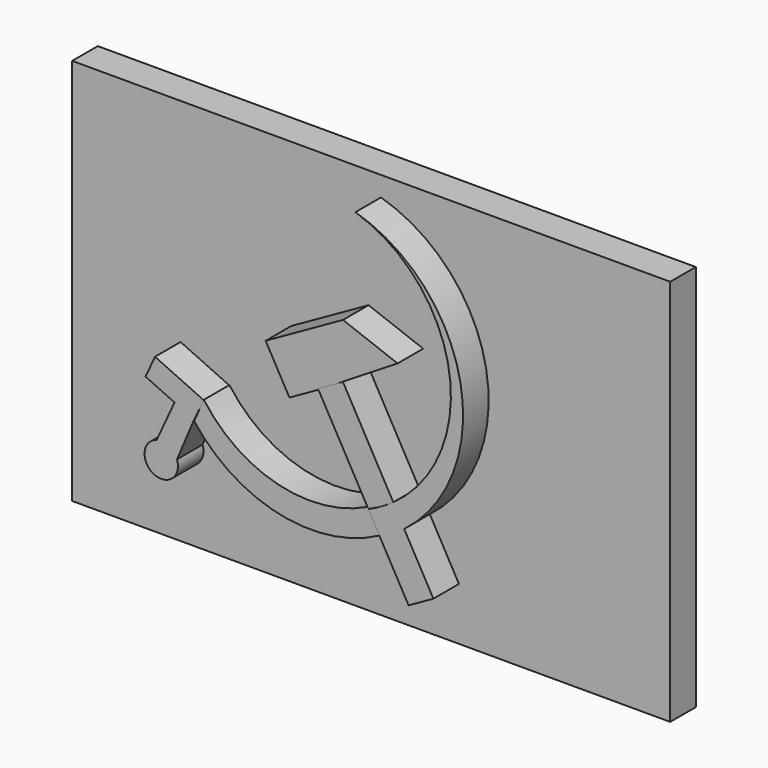
from build123d import *

# Parameters (mm, degrees)
F2_DEPTH = 25.4
F3_W     = 237.6009970903
F3_H     = 153.9654433727
F4_DEPTH = 12.7


with BuildPart() as f2:
    # F0 (on Front) → F2 (new body)
    with BuildSketch(Plane.XZ):
        with BuildLine():
            Line((-64.3306672573, 0), (-71.4252218604, -15.4237253591))
            ThreePointArc((-71.4252218604, -15.4237253591), (-72.6511323462, -27.7185305075), (-63.3521154523, -19.5825994015))
            Line((-63.3521154523, -19.5825994015), (-56.7466728389, -3.9256610908))
            Line((-56.7466728389, -3.9256610908), (-64.3306672573, 0))
        make_face()
        Polygon((-75.8445660615, 5.296125408), (-64.3306672573, 0), (-56.7466728389, -3.9256610908), (-52.6234121387, 4.5160594285), (-72.0855967984, 13.4682112951), align=None)
    extrude(amount=F2_DEPTH)


with BuildPart() as f2b:
    # F0 (on Front) → F2, piece 2 (new body)
    with BuildSketch(Plane.XZ):
        Polygon((-18.6845945711, 16.555041561), (-7.1953465231, 23.0153091252), (24.2997054011, 42.4743108451), (2.6012415412, 50.6354220424), (-28.1310292188, 33.355031617), align=None)
    extrude(amount=F2_DEPTH)


with BuildPart() as f2c:
    # F0 (on Front) → F2, piece 3 (new body)
    with BuildSketch(Plane.XZ):
        with BuildLine():
            ThreePointArc((22.4944953294, -6.7063916159), (17.7171299982, -9.748369789), (12.6509112915, -12.2802226143))
            Line((12.6509112915, -12.2802226143), (17.3099082645, -20.5660051064))
            ThreePointArc((17.3099082645, -20.5660051064), (22.2566100758, -17.7984094918), (26.9180159505, -14.5733917296))
            Line((26.9180159505, -14.5733917296), (22.4944953294, -6.7063916159))
        make_face()
        with BuildLine():
            ThreePointArc((7.5516351178, 89.9414640887), (44.8309857608, 46.2261805414), (22.4944953294, -6.7063916159))
            Line((22.4944953294, -6.7063916159), (26.9180159505, -14.5733917296))
            ThreePointArc((26.9180159505, -14.5733917296), (49.3174772695, 43.6288834146), (7.5516351178, 89.9414640887))
        make_face()
        with BuildLine():
            ThreePointArc((26.9180159505, -14.5733917296), (22.2566100758, -17.7984094918), (17.3099082645, -20.5660051064))
            Line((17.3099082645, -20.5660051064), (28.6526773125, -40.7385267317))
            Line((28.6526773125, -40.7385267317), (38.5128803721, -35.1942517944))
            Line((38.5128803721, -35.1942517944), (26.9180159505, -14.5733917296))
        make_face()
    extrude(amount=F2_DEPTH)


with BuildPart() as f2d:
    # F1 (on Front) → F2, piece 4 (new body)
    with BuildSketch(Plane.XZ):
        with BuildLine():
            Line((-52.6955723763, 4.7223349102), (-56.5307512879, -3.9707440883))
            ThreePointArc((-56.5307512879, -3.9707440883), (-22.6661115444, -25.5245276399), (17.104735598, -20.0785081834))
            Line((17.104735598, -20.0785081834), (12.6471872308, -12.1466942847))
            Line((12.6471872308, -12.1466942847), (12.3380959022, -11.5966935457))
            ThreePointArc((12.3380959022, -11.5966935457), (-23.156184417, -15.3027292619), (-52.6955723763, 4.7223349102))
        make_face()
        with BuildLine():
            Line((12.3380959022, -11.5966935457), (12.6471872308, -12.1466942847))
            ThreePointArc((12.6471872308, -12.1466942847), (17.7628642759, -9.6566366334), (22.6099974974, -6.6774021226))
            Line((22.6099974974, -6.6774021226), (2.5890725665, 28.9480667561))
            Line((2.5890725665, 28.9480667561), (-7.3183678898, 23.3802489035))
            Line((-7.3183678898, 23.3802489035), (12.3380959022, -11.5966935457))
        make_face()
    extrude(amount=F2_DEPTH)


with BuildPart() as f4:
    # F3 (on Front) → F4 (new body)
    with BuildSketch(Plane.XZ):
        with Locations((3.6535635591, 20.8210796118)):
            Rectangle(F3_W, F3_H)
    extrude(amount=F4_DEPTH)


solid = Compound([f2.part, f2b.part, f2c.part, f2d.part, f4.part])
